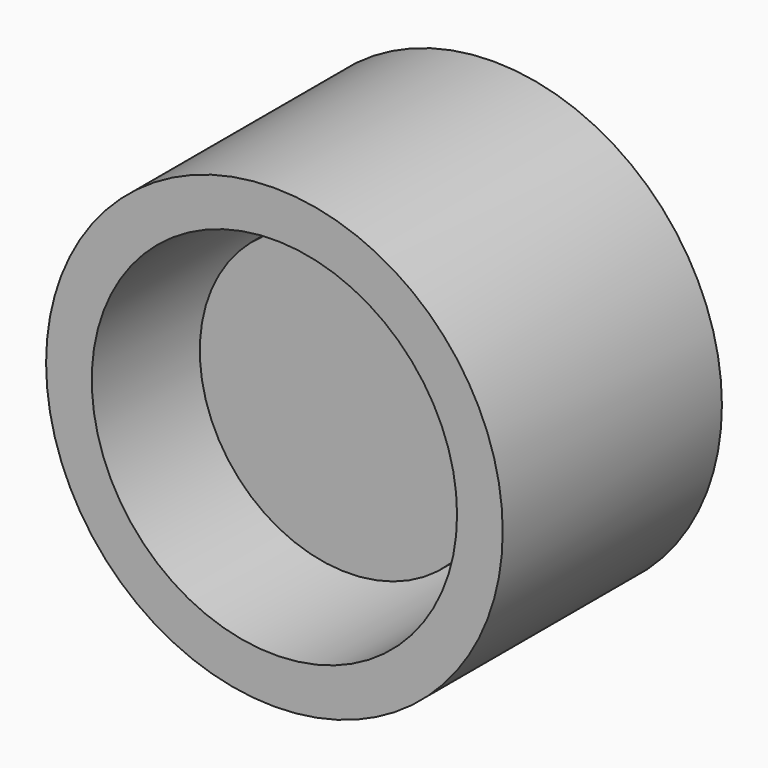
from build123d import *

# Parameters (mm, degrees)
F0_R     = 63.5
F0_R_2   = 50.8
F1_DEPTH = 50.8
F2_W     = 50.8
F2_H     = 50.8
F3_DEPTH = 50.8
F4_R     = 41.0745655778
F5_DEPTH = 25.4
F6_DEPTH = 25.4
F7_DEPTH = 25.4


# Not quite as in the source:
# - a feature names something its author has since deleted; it is built from what else it names


with BuildPart() as f1:
    # F0 (on Front) → F1 (new body)
    with BuildSketch(Plane.XZ):
        Circle(F0_R)
        Circle(F0_R_2, mode=Mode.SUBTRACT)
    extrude(amount=F1_DEPTH)

    # F6 (add): a face of the model
    f6_faces = [f1.faces().sort_by_distance(p)[0] for p in [
        (-61.7039487758, -50.8, 0),
    ]]
    extrude(f6_faces, amount=F6_DEPTH)


with BuildPart() as f3:
    # F2 (on Front) → F3 (new body)
    with BuildSketch(Plane.XZ):
        Rectangle(F2_W, F2_H)
    extrude(amount=F3_DEPTH)

    # F4 (on Front) → F5 (join)
    with BuildSketch(Plane.XZ):
        Circle(F4_R)
    extrude(amount=F5_DEPTH)

    # F7 (add): a face of the model
    f7_faces = [f3.faces().sort_by_distance(p)[0] for p in [
        (-39.9128014236, -25.4, 0),
    ]]
    extrude(f7_faces, amount=F7_DEPTH)


solid = Compound([f1.part, f3.part])
